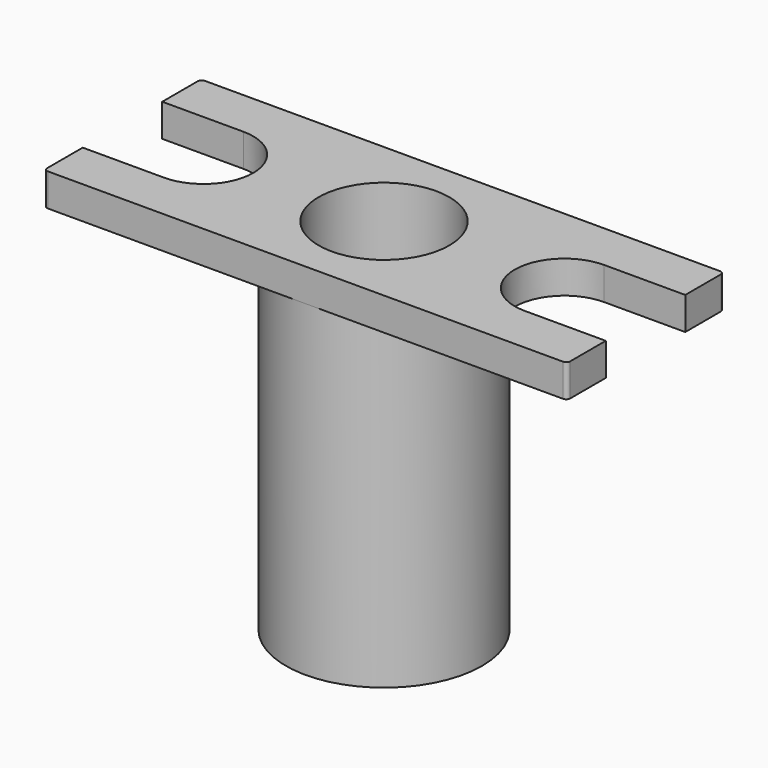
from build123d import *

# Parameters (mm, degrees)
F0_R     = 12.7
F1_DEPTH = 6.35
F2_DEPTH = 63.5
F3_DEPTH = 57.15
F4_R     = 4.7625
F5_DEPTH = 6.35


with BuildPart() as f1:
    # F0 (on Top) → F1 (new body)
    with BuildSketch(Plane.XY):
        with BuildLine():
            Line((3.68e-08, -19.05), (50.038, -19.05))
            ThreePointArc((50.038, -19.05), (50.5768153673, -18.8268153673), (50.8, -18.288))
            Line((50.8, -18.288), (50.8, -9.652))
            Line((50.8, -9.652), (35.052, -9.652))
            ThreePointArc((35.052, -9.652), (25.4, 0), (35.052, 9.652))
            Line((35.052, 9.652), (50.8, 9.652))
            Line((50.8, 9.652), (50.8, 18.288))
            ThreePointArc((50.8, 18.288), (50.5768153673, 18.8268153673), (50.038, 19.05))
            Line((50.038, 19.05), (3.68e-08, 19.05))
            ThreePointArc((3.68e-08, 19.05), (13.4703841946, 13.4703841686), (19.05, 0))
            ThreePointArc((19.05, 0), (13.4703841946, -13.4703841686), (3.68e-08, -19.05))
        make_face()
        with BuildLine():
            Line((-50.038, -19.05), (3.68e-08, -19.05))
            ThreePointArc((3.68e-08, -19.05), (-19.05, 0), (3.68e-08, 19.05))
            Line((3.68e-08, 19.05), (-50.038, 19.05))
            ThreePointArc((-50.038, 19.05), (-50.5768153673, 18.8268153673), (-50.8, 18.288))
            Line((-50.8, 18.288), (-50.8, 9.652))
            Line((-50.8, 9.652), (-35.052, 9.652))
            ThreePointArc((-35.052, 9.652), (-25.4, 0), (-35.052, -9.652))
            Line((-35.052, -9.652), (-50.8, -9.652))
            Line((-50.8, -9.652), (-50.8, -18.288))
            ThreePointArc((-50.8, -18.288), (-50.5768153673, -18.8268153673), (-50.038, -19.05))
        make_face()
        with BuildLine():
            ThreePointArc((3.68e-08, 19.05), (-19.05, 0), (3.68e-08, -19.05))
            ThreePointArc((3.68e-08, -19.05), (13.4703841946, -13.4703841686), (19.05, 0))
            ThreePointArc((19.05, 0), (13.4703841946, 13.4703841686), (3.68e-08, 19.05))
        make_face()
        Circle(F0_R, mode=Mode.SUBTRACT)
    extrude(amount=F1_DEPTH)

    # F0 (on Top) → F2 (join)
    with BuildSketch(Plane.XY):
        with BuildLine():
            ThreePointArc((3.68e-08, 19.05), (-19.05, 0), (3.68e-08, -19.05))
            ThreePointArc((3.68e-08, -19.05), (13.4703841946, -13.4703841686), (19.05, 0))
            ThreePointArc((19.05, 0), (13.4703841946, 13.4703841686), (3.68e-08, 19.05))
        make_face()
        Circle(F0_R, mode=Mode.SUBTRACT)
        Circle(F0_R)
    extrude(amount=-F2_DEPTH)

    # F3 (cut): a face of the model
    f3_faces = [f1.faces().sort_by_distance(p)[0] for p in [
        (0, 0, 0),
    ]]
    extrude(f3_faces, amount=-F3_DEPTH, mode=Mode.SUBTRACT)

    # F4 (on face) → F5 (cut)
    with BuildSketch(Plane(origin=(0, 0, -63.5), x_dir=(1, 0, 0), z_dir=(0, 0, -1))):
        Circle(F4_R)
    extrude(amount=-F5_DEPTH, mode=Mode.SUBTRACT)


solid = f1.part
